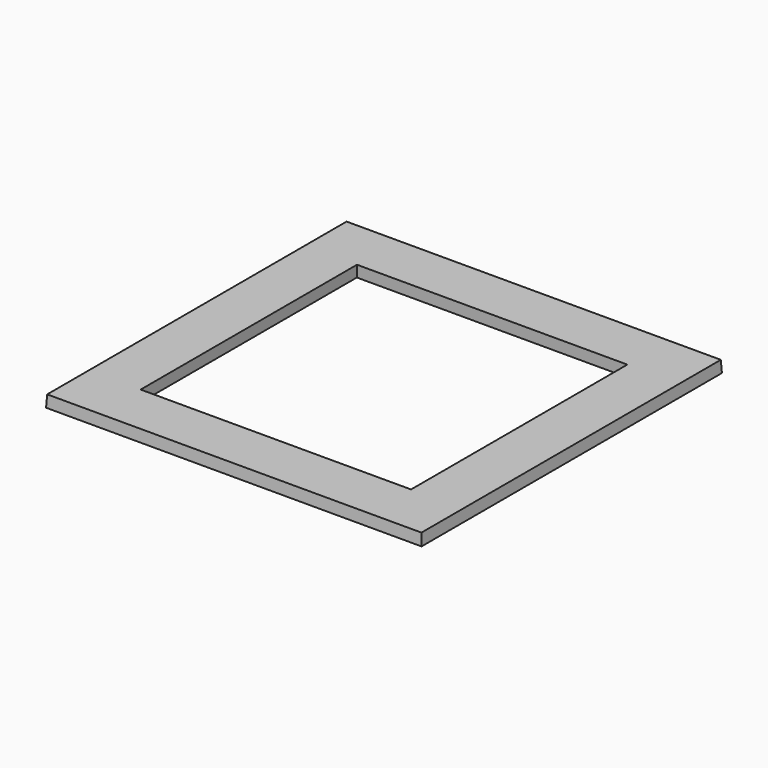
from build123d import *

# Parameters (mm, degrees)
F0_W     = 101.6
F0_H     = 101.6
F1_DEPTH = 3.175
F1_TAPER = 3
F2_T     = -14.0335


# Not quite as in the source:
# - a feature of the source that left no trace in its solid (it failed there, or was rolled back) is left out


with BuildPart() as f1:
    # F0 (on Top) → F1 (new body)
    with BuildSketch(Plane.XY):
        Rectangle(F0_W, F0_H)
    extrude(amount=F1_DEPTH, taper=F1_TAPER)

    # F2
    f2_openings = [f1.faces().sort_by_distance(p)[0] for p in [
        (0, 0, 3.175),
        (0, 0, 0),
    ]]
    offset(amount=F2_T, openings=f2_openings)


solid = f1.part
